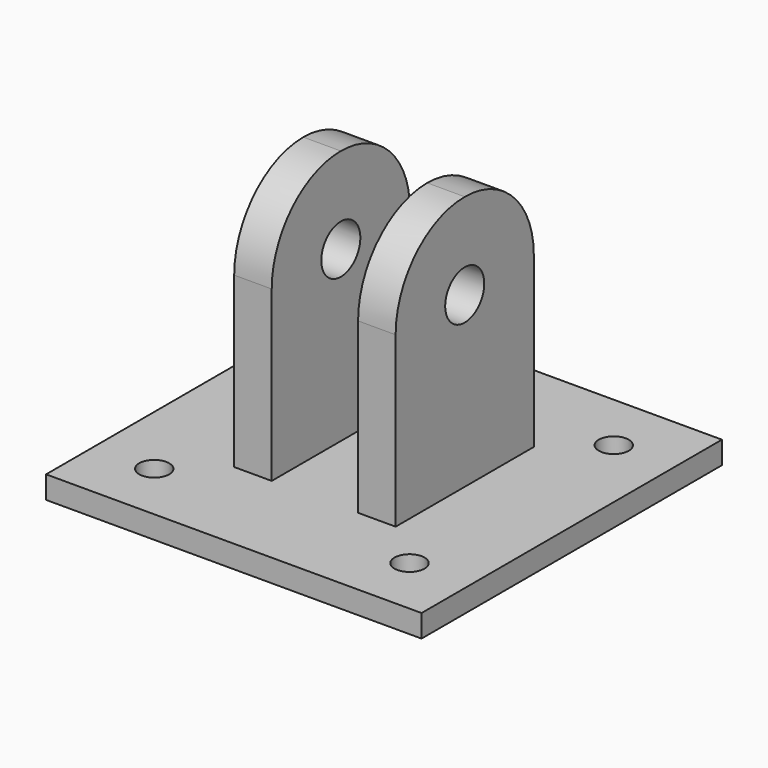
from build123d import *

# Parameters (mm, degrees)
F0_W     = 50
F0_H     = 50
F1_DEPTH = 3
F3_DEPTH = 34
F4_R     = 11.49999
F6_D     = 6.5
F8_D     = 4
F8_DEPTH = 15
F8_TIP   = 1.2017212381


# Not quite as in the source:
# - a fillet or chamfer is up to 0.001 mm smaller than in the source, because OpenCascade refuses the exact size


with BuildPart() as f1:
    # F0 (on Top) → F1 (new body)
    with BuildSketch(Plane.XY):
        Rectangle(F0_W, F0_H)
    extrude(amount=F1_DEPTH)

    # F2 (on face) → F3 (join)
    with BuildSketch(Plane.XY.offset(3)):
        Polygon((5.74977943, 11.5), (5.74977943, 0), (5.74977943, -11.4999999979), (10.74977943, -11.4999999979), (10.74977943, 2.1e-09), (10.74977943, 11.5), align=None)
        Polygon((-5.75022057, -11.4999999979), (-5.75, 0), (-5.74977943, 11.5000000021), (-10.75022057, 11.5000000021), (-10.75022057, 2.1e-09), (-10.75022057, -11.4999999979), align=None)
    extrude(amount=F3_DEPTH)

    # F4 (radius 11.5 in the source; OpenCascade refuses exactly that, so slightly less here)
    f4_edges = [f1.edges().sort_by_distance(p)[0] for p in [
        (-8.250221, -11.5, 37),
        (8.249779, -11.5, 37),
        (8.249779, 11.5, 37),
        (-8.25, 11.5, 37),
    ]]
    fillet(f4_edges, radius=F4_R)

    # F6 (through all)
    with Locations(Plane(origin=(-10.75022057, 0, 0), x_dir=(0, -1, 0), z_dir=(-1, 0, 0))):
        with Locations((-2.1e-09, 25.5)):
            Hole(F6_D / 2)

    # F8
    with Locations(Plane.XY.offset(3)):
        with Locations((-17, 17), (17, 17), (17, -17), (-17, -17)):
            Hole(F8_D / 2, depth=F8_DEPTH)
            with Locations((0, 0, -(F8_DEPTH + F8_TIP / 2))):  # 118° drill point
                Cone(0, F8_D / 2, F8_TIP, mode=Mode.SUBTRACT)


solid = f1.part
